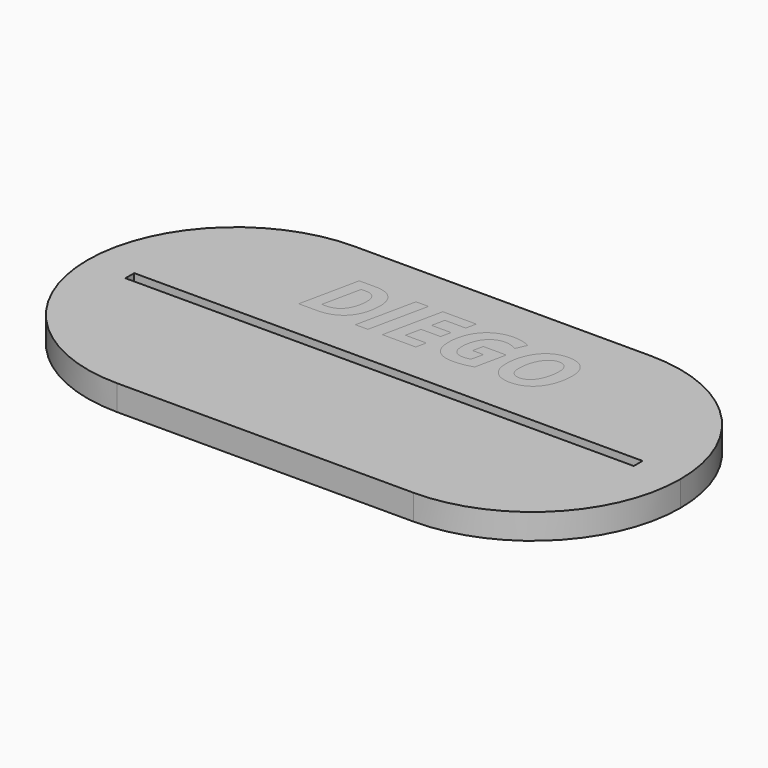
from build123d import *

# Parameters (mm, degrees)
F0_W         = 70
F0_H         = 35
F0_W_2       = 60
F0_H_2       = 1.3
F1_DEPTH     = 3
F2_R         = 17.49999
F3_SIZE      = 1
F4_TEXT_SIZE = 9.8863564846
F5_DEPTH     = 1.5


# Not quite as in the source:
# - a fillet or chamfer is up to 0.001 mm smaller than in the source, because OpenCascade refuses the exact size
# - Text() gives the source's letters only with a copy of the font that has no kerning and outlines rounded to 1/6400 em; it was checked with that copy


with BuildPart() as f1:
    # F0 (on Top) → F1 (new body)
    with BuildSketch(Plane.XY):
        with Locations((35, 17.5)):
            Rectangle(F0_W, F0_H)
        with Locations((35, 17.5)):
            Rectangle(F0_W_2, F0_H_2, mode=Mode.SUBTRACT)
    extrude(amount=F1_DEPTH)

    # F2 (radius 17.5 in the source; OpenCascade refuses exactly that, so slightly less here)
    f2_edges = [f1.edges().sort_by_distance(p)[0] for p in [
        (70, 0, 1.5),
        (70, 35, 1.5),
        (0, 35, 1.5),
        (0, 0, 1.5),
    ]]
    fillet(f2_edges, radius=F2_R)

    # F3
    f3_edges = [f1.edges().sort_by_distance(p)[0] for p in [
        (35, 16.85, 0),
        (35, 18.15, 0),
    ]]
    chamfer(f3_edges, length=F3_SIZE)


with BuildPart() as f5:
    # F4 (on face) → F5 (new body)
    with BuildSketch(Plane.XY.offset(3)):
        with Locations((20.4017814249, 22.8461325169)):
            Text('DIEGO', F4_TEXT_SIZE, font='Open Sans', font_style=FontStyle.BOLDITALIC, text_align=(TextAlign.LEFT, TextAlign.BOTTOM))
    extrude(amount=-F5_DEPTH)


solid = Compound([f1.part, f5.part])
